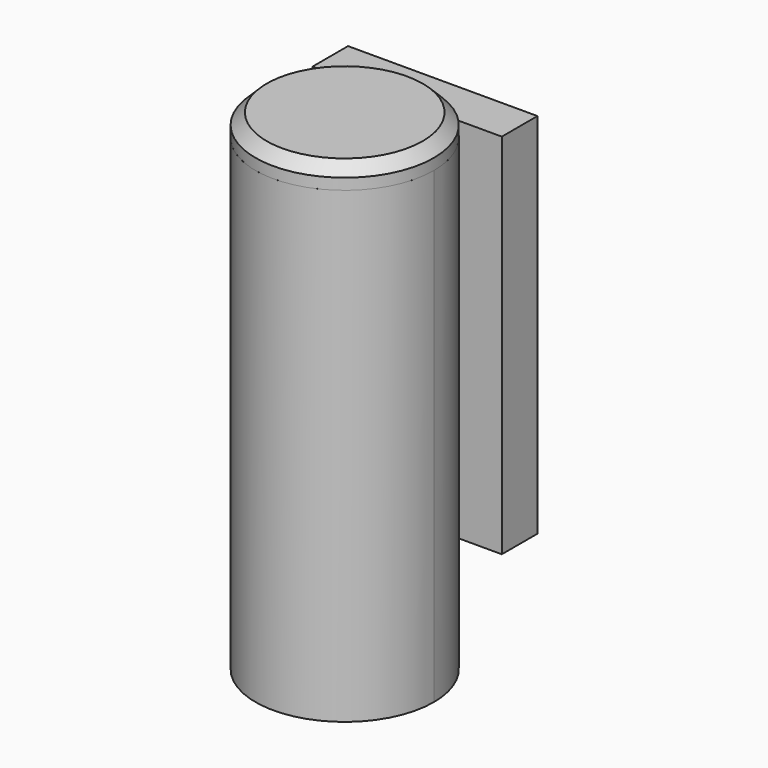
from build123d import *

# Parameters (mm, degrees)
F0_W      = 17
F0_H      = 33
F0_R      = 2.5
F0_R_2    = 1
F1_DEPTH  = 4
F3_DEPTH  = 33
F4_R      = 6.5
F5_DEPTH  = 42
F6_R      = 1
F7_DEPTH  = 1
F8_R      = 6.5
F9_DEPTH  = 4
F8_R_2    = 8
F10_DEPTH = 2
F11_SIZE  = 1


with BuildPart() as f1:
    # F0 (on Front) → F1 (new body)
    with BuildSketch(Plane.XZ):
        with Locations((8.5, 16.5)):
            Rectangle(F0_W, F0_H)
        with Locations((8.5, 16)):
            Circle(F0_R, mode=Mode.SUBTRACT)
        with Locations((8.5, 29)):
            Circle(F0_R_2, mode=Mode.SUBTRACT)
    extrude(amount=F1_DEPTH)

    # F2 (on face) → F3 (cut, through all)
    with BuildSketch(Plane(origin=(0, 0, 0), x_dir=(1, 0, 0), z_dir=(0, 0, -1))):
        with BuildLine():
            ThreePointArc((4.6270166538, 4), (6.5, 3.2540333076), (8.5, 3))
            ThreePointArc((8.5, 3), (10.5, 3.2540333076), (12.3729833462, 4))
            Line((12.3729833462, 4), (4.6270166538, 4))
        make_face()
    extrude(amount=-F3_DEPTH, mode=Mode.SUBTRACT)


with BuildPart() as f5:
    # F4 (on face) → F5 (new body)
    with BuildSketch(Plane.XY.offset(33)):
        with BuildLine():
            ThreePointArc((12.3729833462, -4), (8.5, -3), (4.6270166538, -4))
            ThreePointArc((4.6270166538, -4), (4.4369879873, -17.8914391374), (16.5, -11))
            ThreePointArc((16.5, -11), (15.3914391374, -6.9369879873), (12.3729833462, -4))
        make_face()
        with Locations((8.5, -11)):
            Circle(F4_R, mode=Mode.SUBTRACT)
    extrude(amount=-F5_DEPTH)

    # F6 (on face) → F7 (cut, symmetric)
    with BuildSketch(Plane.XZ.offset(4)):
        with Locations((8.5, 29)):
            Circle(F6_R)
    extrude(amount=F7_DEPTH, both=True, mode=Mode.SUBTRACT)


with BuildPart() as f9:
    # F8 (on face) → F9 (new body)
    with BuildSketch(Plane.XY.offset(33)):
        with Locations((8.5, -11)):
            Circle(F8_R)
    extrude(amount=-F9_DEPTH)

    # F8 (on face) → F10 (join)
    with BuildSketch(Plane.XY.offset(33)):
        with Locations((8.5, -11)):
            Circle(F8_R_2)
        with Locations((8.5, -11)):
            Circle(F8_R, mode=Mode.SUBTRACT)
        with Locations((8.5, -11)):
            Circle(F8_R)
    extrude(amount=F10_DEPTH)

    # F11
    f11_edges = [f9.edges().sort_by_distance(p)[0] for p in [
        (0.5, -11, 35),
    ]]
    chamfer(f11_edges, length=F11_SIZE)


solid = Compound([f1.part, f5.part, f9.part])
